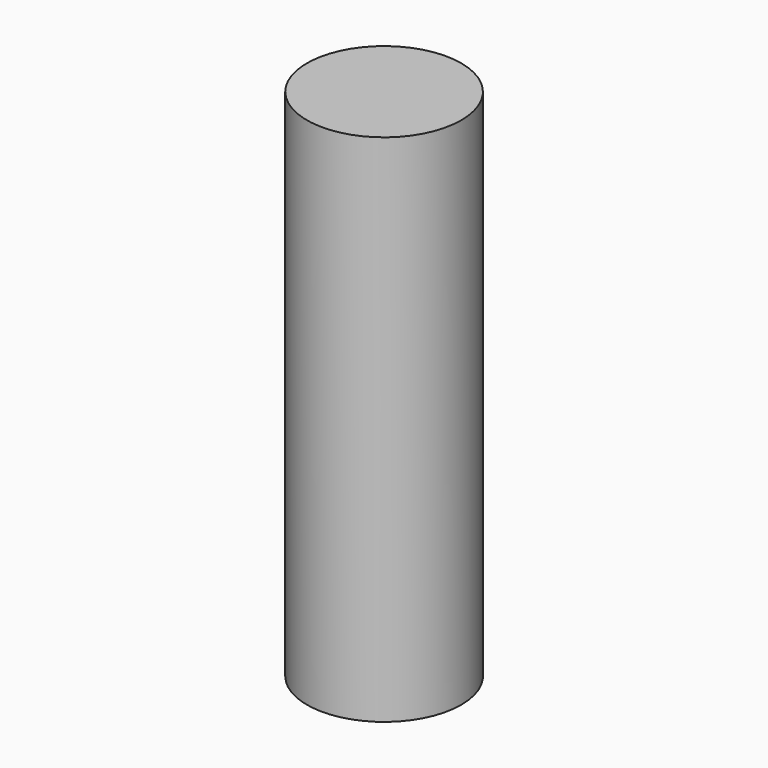
from build123d import *

# Parameters (mm, degrees)
F0_R     = 7.5
F1_DEPTH = 50


# Not quite as in the source:
# - a feature of the source that left no trace in its solid (it failed there, or was rolled back) is left out


with BuildPart() as f1:
    # F0 (on Top) → F1 (new body)
    with BuildSketch(Plane.XY):
        Circle(F0_R)
    extrude(amount=F1_DEPTH)


solid = f1.part
